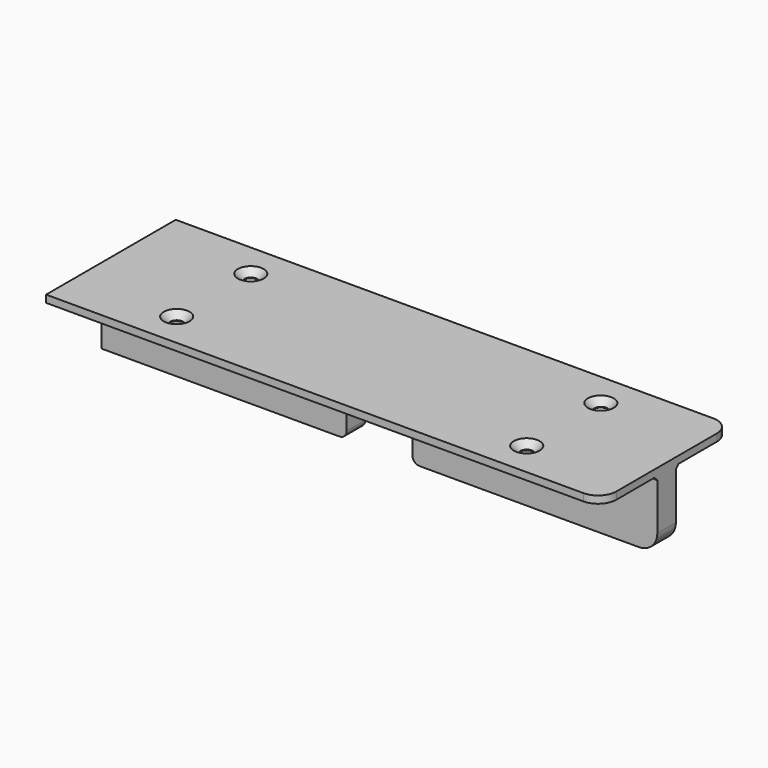
from build123d import *

# Parameters (mm, degrees)
F0_W         = 152.4
F0_H         = 44.45
F1_DEPTH     = 2
F2_W         = 152.4
F2_H         = 6.35
F3_DEPTH     = 18.796
F4_R         = 1.75
F5_DEPTH     = 25
F7_DEPTH     = 25.401
F8_SIZE      = 1.8
F9_T4_DEPTH  = 152.4
F9_S5_R      = 9
F9_T6_DEPTH  = 78
F9_T10_DEPTH = 152.4
F9_S11_R     = 9
F9_T12_DEPTH = 78
F10_R        = 2
F11_R        = 5


# Not quite as in the source:
# - a fillet or chamfer that OpenCascade refuses, or shapes differently, is made with other operations: its cross-section is extruded or revolved along the edge and cut away or added
# - a feature names something its author has since deleted; it is built from what else it names


with BuildPart() as f1:
    # F0 (on Top) → F1 (new body)
    with BuildSketch(Plane.XY):
        Rectangle(F0_W, F0_H)
    extrude(amount=F1_DEPTH)

    # F2 (on face) → F3 (join)
    with BuildSketch(Plane(origin=(0, 0, 0), x_dir=(1, 0, 0), z_dir=(0, 0, -1))):
        Rectangle(F2_W, F2_H)
    extrude(amount=F3_DEPTH)

    # F4 (on face) → F5 (cut)
    with BuildSketch(Plane(origin=(0, 0, 0), x_dir=(1, 0, 0), z_dir=(0, 0, -1))):
        with Locations((48, -12.7)):
            Circle(F4_R)
        with Locations((-48, -12.7)):
            Circle(F4_R)
        with Locations((-48, 12.7)):
            Circle(F4_R)
        with Locations((48, 12.7)):
            Circle(F4_R)
    extrude(amount=-F5_DEPTH, mode=Mode.SUBTRACT)

    # F6 (on face) → F7 (cut, through all)
    with BuildSketch(Plane(origin=(0, 3.175, 0), x_dir=(-1, 0, 0), z_dir=(0, 1, 0))):
        with BuildLine():
            ThreePointArc((-9, -9.398), (0, -18.398), (9, -9.398))
            ThreePointArc((9, -9.398), (0, -0.398), (-9, -9.398))
        make_face()
        with BuildLine():
            Line((9, -18.796), (9, -9.398))
            ThreePointArc((9, -9.398), (0, -18.398), (-9, -9.398))
            Line((-9, -9.398), (-9, -18.796))
            Line((-9, -18.796), (9, -18.796))
        make_face()
    extrude(amount=-F7_DEPTH, mode=Mode.SUBTRACT)

    # F8
    f8_edges = [f1.edges().sort_by_distance(p)[0] for p in [
        (46.25, -12.7, 2),
        (-49.75, -12.7, 2),
        (-49.75, 12.7, 2),
        (46.25, 12.7, 2),
    ]]
    chamfer(f8_edges, length=F8_SIZE)

    # F9: chamfer of 1 on 2 edges, made by hand


with BuildPart() as f9_tool2:
    # F9_s3 → F9_t4 (new body)
    with BuildSketch(Plane.YZ.offset(-76.2)):
        Polygon((3.175, -1), (4.175, 0), (3.175, 0), align=None)
    extrude(amount=F9_T4_DEPTH)

    # F9_s5 → F9_t6 (cut, symmetric)
    with BuildSketch(Plane.XZ.offset(-3.7)):
        with Locations((0, -9.398)):
            Circle(F9_S5_R)
    extrude(amount=F9_T6_DEPTH, both=True, mode=Mode.SUBTRACT)


with BuildPart() as f1_1:
    add(f1.part)

    # F9_t1: union F9_tool2
    add(f9_tool2.part)


with BuildPart() as f9_tool8:
    # F9_s9 → F9_t10 (new body)
    with BuildSketch(Plane.YZ.offset(76.2)):
        Polygon((-4.175, 0), (-3.175, -1), (-3.175, 0), align=None)
    extrude(amount=-F9_T10_DEPTH)

    # F9_s11 → F9_t12 (cut, symmetric)
    with BuildSketch(Plane.XZ.offset(3.7)):
        with Locations((0, -9.398)):
            Circle(F9_S11_R)
    extrude(amount=F9_T12_DEPTH, both=True, mode=Mode.SUBTRACT)


with BuildPart() as f1_2:
    add(f1_1.part)

    # F9_t7: union F9_tool8
    add(f9_tool8.part)

    # F10
    f10_edges = [f1_2.edges().sort_by_distance(p)[0] for p in [
        (9, 0, -18.796),
        (-9, 0, -18.796),
    ]]
    fillet(f10_edges, radius=F10_R)

    # F11
    f11_edges = [f1_2.edges().sort_by_distance(p)[0] for p in [
        (76.2, 0, -18.796),
        (76.2, -22.225, 1),
        (76.2, 22.225, 1),
    ]]
    fillet(f11_edges, radius=F11_R)


solid = f1_2.part
